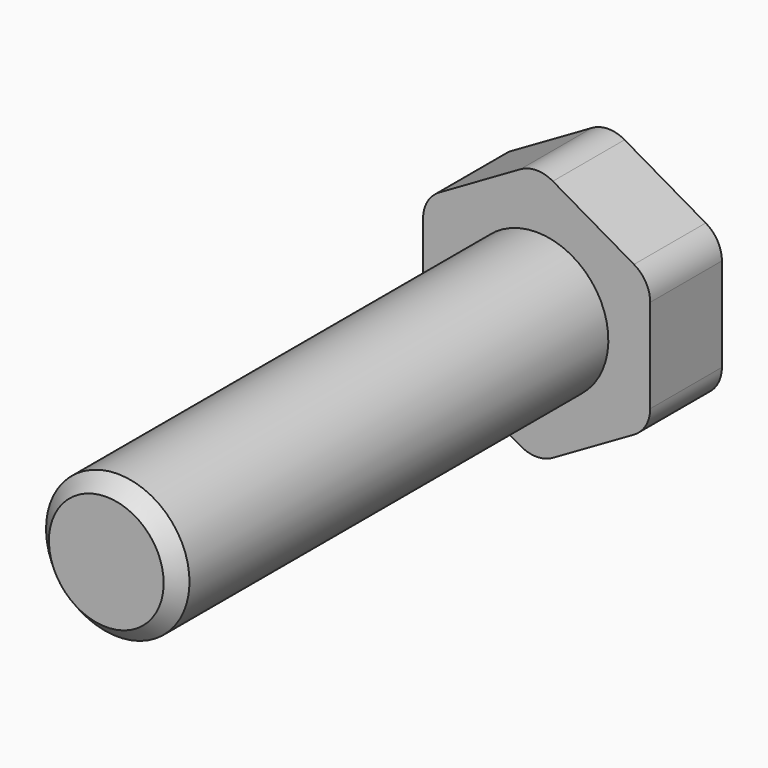
from build123d import *

# Parameters (mm, degrees)
F2_R     = 15.825
F3_DEPTH = 25


# Not quite as in the source:
# - a feature names something its author has since deleted; it is built from what else it names


with BuildPart() as f1:
    # F0 (on Right) → F1 (revolve)
    with BuildSketch(Plane.YZ):
        Polygon((0, 15.825), (0, 6), (-43.8, 6), (-45, 4.8), (-45, 0), (7.5, 0), (7.5, 15.825), align=None)
    revolve(axis=Axis((0, -18.75, 0), (0, -1, 0)))

    # F2 (on face) → F3 (cut)
    with BuildSketch(Plane(origin=(0, 7.5, 0), x_dir=(-1, 0, 0), z_dir=(0, 1, 0))):
        Circle(F2_R)
        with BuildLine():
            ThreePointArc((1.3563466521, -10.1865680099), (0, -10.55), (-1.3563466521, -10.1865680099))
            Line((-1.3563466521, -10.1865680099), (-8.1436533479, -6.267914662))
            ThreePointArc((-8.1436533479, -6.267914662), (-9.1365680099, -5.275), (-9.5, -3.9186533479))
            Line((-9.5, -3.9186533479), (-9.5, 3.9186533479))
            ThreePointArc((-9.5, 3.9186533479), (-9.1365680099, 5.275), (-8.1436533479, 6.267914662))
            Line((-8.1436533479, 6.267914662), (-1.3563466521, 10.1865680099))
            ThreePointArc((-1.3563466521, 10.1865680099), (0, 10.55), (1.3563466521, 10.1865680099))
            Line((1.3563466521, 10.1865680099), (8.1436533479, 6.267914662))
            ThreePointArc((8.1436533479, 6.267914662), (9.1365680099, 5.275), (9.5, 3.9186533479))
            Line((9.5, 3.9186533479), (9.5, -3.9186533479))
            ThreePointArc((9.5, -3.9186533479), (9.1365680099, -5.275), (8.1436533479, -6.267914662))
            Line((8.1436533479, -6.267914662), (1.3563466521, -10.1865680099))
        make_face(mode=Mode.SUBTRACT)
    extrude(amount=-F3_DEPTH, mode=Mode.SUBTRACT)


solid = f1.part
